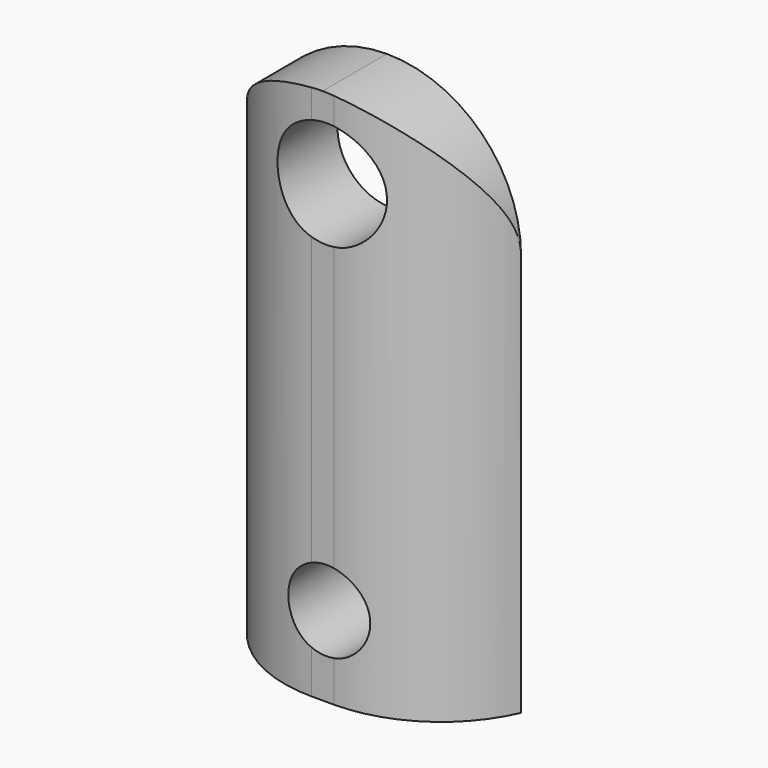
from build123d import *

# Parameters (mm, degrees)
F0_W        = 10
F0_H        = 20
F1_DEPTH    = 3
F2_R        = 2
F2_R_2      = 1.5
F3_DEPTH    = 3.001
F4_T1_DEPTH = 28
F4_T3_DEPTH = 42.9128784748


# Not quite as in the source:
# - a fillet or chamfer that OpenCascade refuses, or shapes differently, is made with other operations: its cross-section is extruded or revolved along the edge and cut away or added


with BuildPart() as f1:
    # F0 (on Front) → F1 (new body)
    with BuildSketch(Plane.XZ):
        with Locations((-0.1535092495, 0.14802441)):
            Rectangle(F0_W, F0_H)
    extrude(amount=F1_DEPTH)

    # F2 (on face) → F3 (cut, through all)
    with BuildSketch(Plane.XZ.offset(3)):
        with Locations((0, 7.14802441)):
            Circle(F2_R)
        with Locations((0, -6.85197559)):
            Circle(F2_R_2)
    extrude(amount=-F3_DEPTH, mode=Mode.SUBTRACT)

    # F4: fillet of radius 5 on 4 edges, made by hand

    # F4_s2 → F4_t1 (cut)
    with BuildSketch(Plane.XZ.offset(-12.5)):
        with BuildLine():
            ThreePointArc((4.8464907505, 5.14802441), (3.3820246565, 8.6835583159), (-0.1535092495, 10.14802441))
            Line((-0.1535092495, 10.14802441), (4.8464907505, 10.14802441))
            Line((4.8464907505, 10.14802441), (4.8464907505, 5.14802441))
        make_face()
        with BuildLine():
            ThreePointArc((-5.1535092495, 5.14802441), (-3.6890431554, 8.6835583159), (-0.1535092495, 10.14802441))
            Line((-0.1535092495, 10.14802441), (-5.1535092495, 10.14802441))
            Line((-5.1535092495, 10.14802441), (-5.1535092495, 5.14802441))
        make_face()
    extrude(amount=F4_T1_DEPTH, mode=Mode.SUBTRACT)

    # F4_s4 → F4_t3 (cut)
    with BuildSketch(Plane.XY.offset(-21.3084148274)):
        with BuildLine():
            ThreePointArc((-5.1535092495, 0), (-3.309546342, -2.1833001327), (-0.5709335545, -3))
            Line((-0.5709335545, -3), (-5.1535092495, -3))
            Line((-5.1535092495, -3), (-5.1535092495, 0))
        make_face()
        with BuildLine():
            ThreePointArc((4.8464907505, 0), (3.0025278431, -2.1833001327), (0.2639150556, -3))
            Line((0.2639150556, -3), (4.8464907505, -3))
            Line((4.8464907505, -3), (4.8464907505, 0))
        make_face()
    extrude(amount=F4_T3_DEPTH, mode=Mode.SUBTRACT)


solid = f1.part
